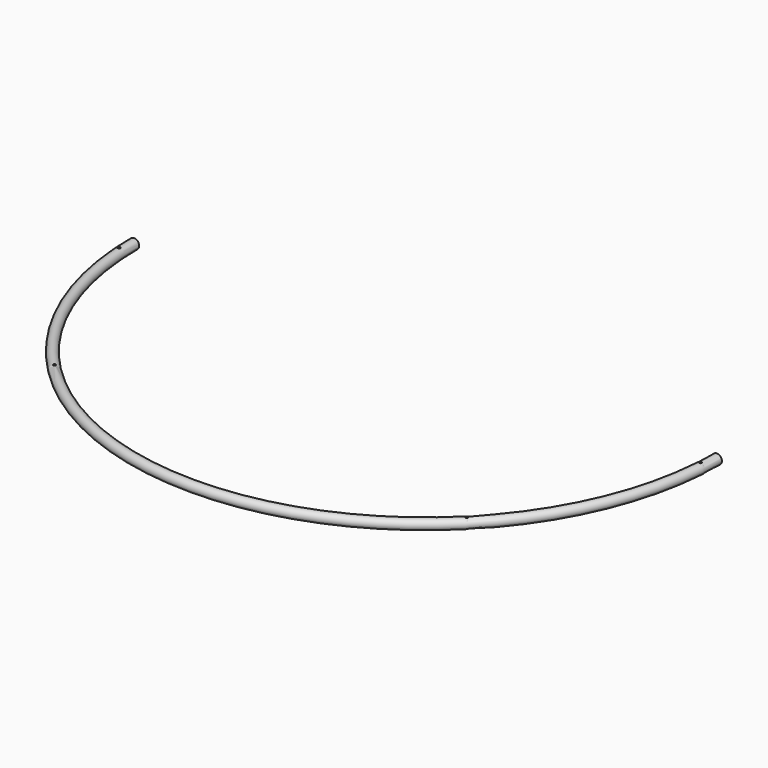
from build123d import *
from build123d import SkipClean  # not in build123d's __all__

# Parameters (mm, degrees)
F0_R          = 19.05
F0_R_2        = 15.85
F1_ANGLE      = 180
F2_R          = 5.25
F3_DEPTH      = 19.0510001
F3_DEPTH_BACK = 19.0510001
F4_R          = 5
F5_DEPTH      = 19.0510001007
F5_DEPTH_BACK = 25


with BuildPart() as f1:
    # F0 (on Front) → F1 (revolve)
    with BuildSketch(Plane.XZ):
        with Locations((-1100, 0)):
            Circle(F0_R)
        with Locations((-1100, 0)):
            Circle(F0_R_2, mode=Mode.SUBTRACT)
    revolve(axis=Axis((0, 0, 190.0846064091), (0, 0, 1)), revolution_arc=F1_ANGLE)

    # F2 (on Top) → F3 (cut, two sides)
    with BuildSketch(Plane.XY) as f3_sk:
        with Locations((-1097.4402033824, -75)):
            Circle(F2_R)
        with Locations((1097.4402033824, -75)):
            Circle(F2_R)
    with SkipClean():  # cleaning this boolean's faces spoils the solid; the shape is the same uncleaned
        extrude(amount=-F3_DEPTH, mode=Mode.SUBTRACT)
        extrude(f3_sk.sketch, amount=F3_DEPTH_BACK, mode=Mode.SUBTRACT)

    # F4 (on Top) → F5 (cut, two sides)
    with BuildSketch(Plane.XY) as f5_sk:
        with Locations((-777.8174593052, -777.8174593052)):
            Circle(F4_R)
        with Locations((777.8174593052, -777.8174593052)):
            Circle(F4_R)
    with SkipClean():  # cleaning this boolean's faces spoils the solid; the shape is the same uncleaned
        extrude(amount=-F5_DEPTH, mode=Mode.SUBTRACT)
        extrude(f5_sk.sketch, amount=F5_DEPTH_BACK, mode=Mode.SUBTRACT)


solid = f1.part
